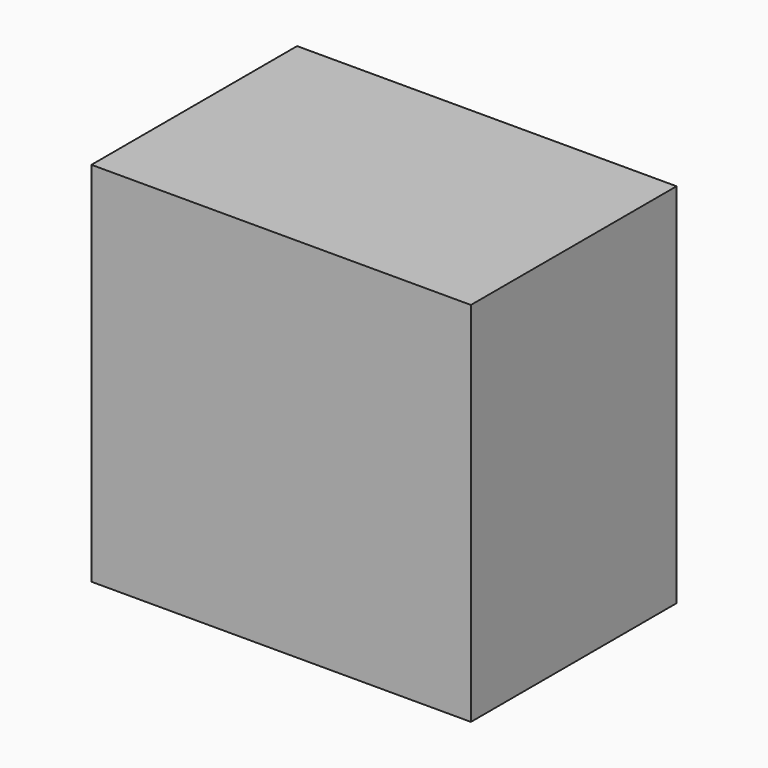
from build123d import *

# Parameters (mm, degrees)
F0_W     = 152.0279198885
F0_H     = 73.5310763121
F1_DEPTH = 102.9895376414


# Not quite as in the source:
# - a feature names something its author has since deleted; it is built from what else it names


with BuildPart() as f1:
    # F0 (on Front) → F1 (new body)
    with BuildSketch(Plane.XZ):
        with Locations((1.0790154338, -36.765538156)):
            Rectangle(F0_W, F0_H)
        with Locations((1.0790154338, 36.765538156)):
            Rectangle(F0_W, F0_H)
    extrude(amount=-F1_DEPTH)


solid = f1.part
